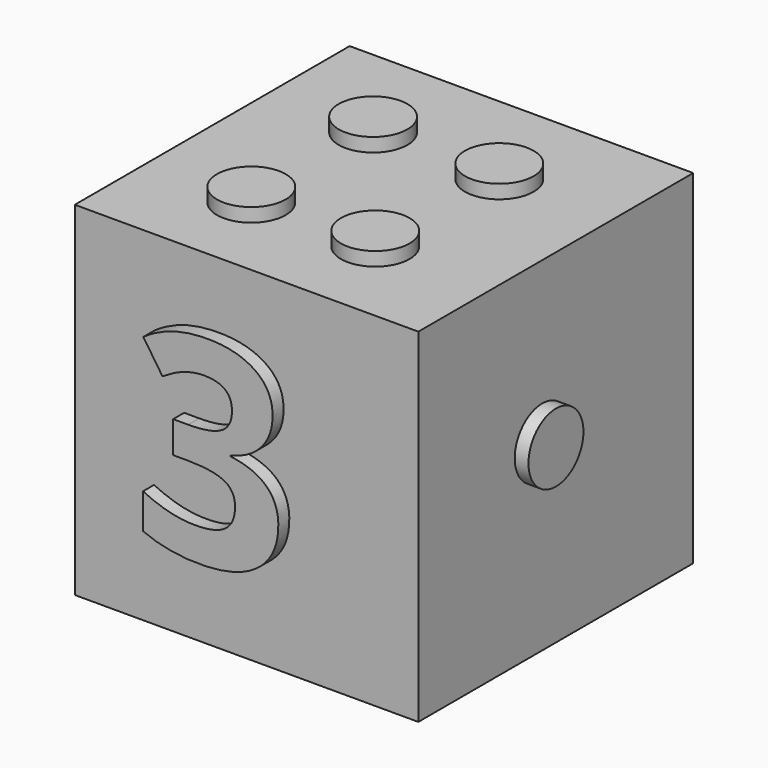
from build123d import *

# Parameters (mm, degrees)
F0_W          = 63.5
F0_H          = 63.5
F1_DEPTH      = 63.5
F6_R          = 6.35
F5_R          = 6.35
F4_R          = 6.35
F3_R          = 6.35
F2_R          = 6.35
F7_DEPTH      = 2.54
F8_TEXT_SIZE  = 50.5958243998
F9_DEPTH      = 2.54
F10_TEXT_SIZE = 47.3323316934
F11_DEPTH     = 2.54
F12_R         = 6.35
F13_DEPTH     = 2.54
F14_TEXT_SIZE = 47.5209736679
F15_DEPTH     = 2.54
F19_R         = 6.35
F18_R         = 6.35
F17_R         = 6.35
F16_R         = 6.35
F20_DEPTH     = 2.54


# Not quite as in the source:
# - Text() gives the source's letters only with a copy of the font that has no kerning and outlines rounded to 1/6400 em; it was checked with that copy


with BuildPart() as f1:
    # F0 (on Front) → F1 (new body)
    with BuildSketch(Plane.XZ):
        with Locations((1.4093826413, -6.4480352104)):
            Rectangle(F0_W, F0_H)
    extrude(amount=F1_DEPTH)

    # F6 (on face) + F5 (on face) + F4 (on face) + F3 (on face) + F2 (on face) → F7 (join)
    with BuildSketch(Plane(origin=(-30.3406173587, 0, 0), x_dir=(0, -1, 0), z_dir=(-1, 0, 0))):
        with Locations((15.0134842843, 12.2437588871)):
            Circle(F6_R)
    with BuildSketch(Plane(origin=(-30.3406173587, 0, 0), x_dir=(0, -1, 0), z_dir=(-1, 0, 0))):
        with Locations((46.5024486184, 12.8694605082)):
            Circle(F5_R)
    with BuildSketch(Plane(origin=(-30.3406173587, 0, 0), x_dir=(0, -1, 0), z_dir=(-1, 0, 0))):
        with Locations((30.4386075586, -6.1582382768)):
            Circle(F4_R)
    with BuildSketch(Plane(origin=(-30.3406173587, 0, 0), x_dir=(0, -1, 0), z_dir=(-1, 0, 0))):
        with Locations((48.3451336622, -23.4257057309)):
            Circle(F3_R)
    with BuildSketch(Plane(origin=(-30.3406173587, 0, 0), x_dir=(0, -1, 0), z_dir=(-1, 0, 0))):
        with Locations((14.7974742576, -23.0567250401)):
            Circle(F2_R)
    extrude(amount=F7_DEPTH)

    # F8 (on face) → F9 (join)
    with BuildSketch(Plane.XZ.offset(63.5)):
        with Locations((-17.6163535798, -23.4719523014)):
            Text('3', F8_TEXT_SIZE, font='Open Sans', font_style=FontStyle.BOLD, text_align=(TextAlign.LEFT, TextAlign.BOTTOM))
    extrude(amount=F9_DEPTH)

    # F10 (on face) → F11 (join)
    with BuildSketch(Plane(origin=(0, 0, 0), x_dir=(-1, 0, 0), z_dir=(0, 1, 0))):
        with Locations((-16.5017300751, -22.1271389164)):
            Text('6', F10_TEXT_SIZE, font='Open Sans', font_style=FontStyle.BOLD, text_align=(TextAlign.LEFT, TextAlign.BOTTOM))
    extrude(amount=F11_DEPTH)

    # F12 (on face) → F13 (join)
    with BuildSketch(Plane.YZ.offset(33.1593826413)):
        with Locations((-34.8878353834, -4.3557123281)):
            Circle(F12_R)
    extrude(amount=F13_DEPTH)

    # F14 (on face) → F15 (join)
    with BuildSketch(Plane(origin=(0, 0, -38.1980352104), x_dir=(1, 0, 0), z_dir=(0, 0, -1))):
        with Locations((-18.2250104845, 15.4068237171)):
            Text('2', F14_TEXT_SIZE, font='Open Sans', font_style=FontStyle.BOLD, text_align=(TextAlign.LEFT, TextAlign.BOTTOM))
    extrude(amount=F15_DEPTH)

    # F19 (on face) + F18 (on face) + F17 (on face) + F16 (on face) → F20 (join)
    with BuildSketch(Plane.XY.offset(25.3019647896)):
        with Locations((12.4927451834, -18.9605727792)):
            Circle(F19_R)
    with BuildSketch(Plane.XY.offset(25.3019647896)):
        with Locations((11.6483019665, -46.5689077973)):
            Circle(F18_R)
    with BuildSketch(Plane.XY.offset(25.3019647896)):
        with Locations((-10.8696185052, -18.9258661121)):
            Circle(F17_R)
    with BuildSketch(Plane.XY.offset(25.3019647896)):
        with Locations((-10.9002171084, -47.0146723092)):
            Circle(F16_R)
    extrude(amount=F20_DEPTH)


solid = f1.part
